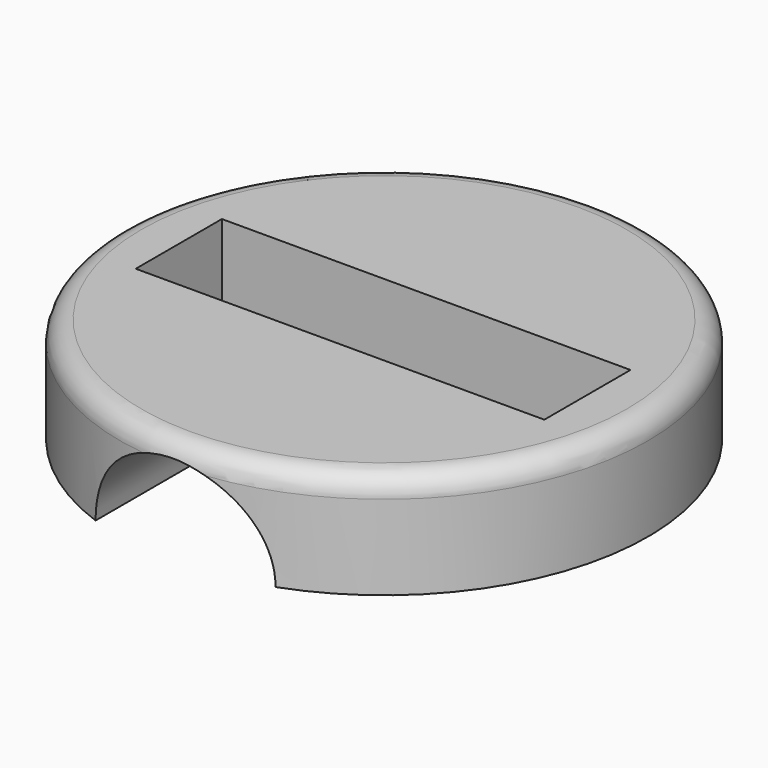
from build123d import *

# Parameters (mm, degrees)
F0_R     = 25
F1_DEPTH = 10
F2_W     = 38.7
F2_H     = 10.2
F3_DEPTH = 11
F4_W     = 10.2
F4_H     = 1.3916883618
F5_DEPTH = 2
F6_W     = 10.2
F6_H     = 1.392
F7_DEPTH = 2
F9_DEPTH = 25


# Not quite as in the source:
# - a fillet or chamfer that OpenCascade refuses, or shapes differently, is made with other operations: its cross-section is extruded or revolved along the edge and cut away or added


with BuildPart() as f1:
    # F0 (on Top) → F1 (new body)
    with BuildSketch(Plane.XY):
        Circle(F0_R)
    extrude(amount=F1_DEPTH)

    # F2 (on face) → F3 (cut)
    with BuildSketch(Plane.XY.offset(10)):
        with Locations((-0.05, -0.05)):
            Rectangle(F2_W, F2_H)
    extrude(amount=-F3_DEPTH, mode=Mode.SUBTRACT)

    # F4 (on face) → F5 (join)
    with BuildSketch(Plane(origin=(19.3, 0, 0), x_dir=(0, -1, 0), z_dir=(-1, 0, 0))):
        with Locations((0.05, 0.6958441809)):
            Rectangle(F4_W, F4_H)
    extrude(amount=F5_DEPTH)

    # F6 (on face) → F7 (join)
    with BuildSketch(Plane.YZ.offset(-19.4)):
        with Locations((-0.05, 0.696)):
            Rectangle(F6_W, F6_H)
    extrude(amount=F7_DEPTH)

    # F8 (on face) → F9 (cut)
    with BuildSketch(Plane(origin=(0, -5.15, 0), x_dir=(-1, 0, 0), z_dir=(0, 1, 0))):
        with BuildLine():
            Line((-8.5235216661, 0), (8.5235216661, 0))
            ThreePointArc((8.5235216661, 0), (0, 8.5235216661), (-8.5235216661, 0))
        make_face()
    extrude(amount=-F9_DEPTH, mode=Mode.SUBTRACT)

    # F10: fillet of radius 2 on 1 edges, made by hand

    # F10_s1 → F10_t2 (revolve, cut)
    with BuildSketch(Plane.XZ):
        with BuildLine():
            ThreePointArc((25, 8), (24.4142135624, 9.4142135624), (23, 10))
            Line((23, 10), (25, 10))
            Line((25, 10), (25, 8))
        make_face()
    revolve(axis=Axis((0, 0, 10), (0, 0, 1)), mode=Mode.SUBTRACT)


solid = f1.part
